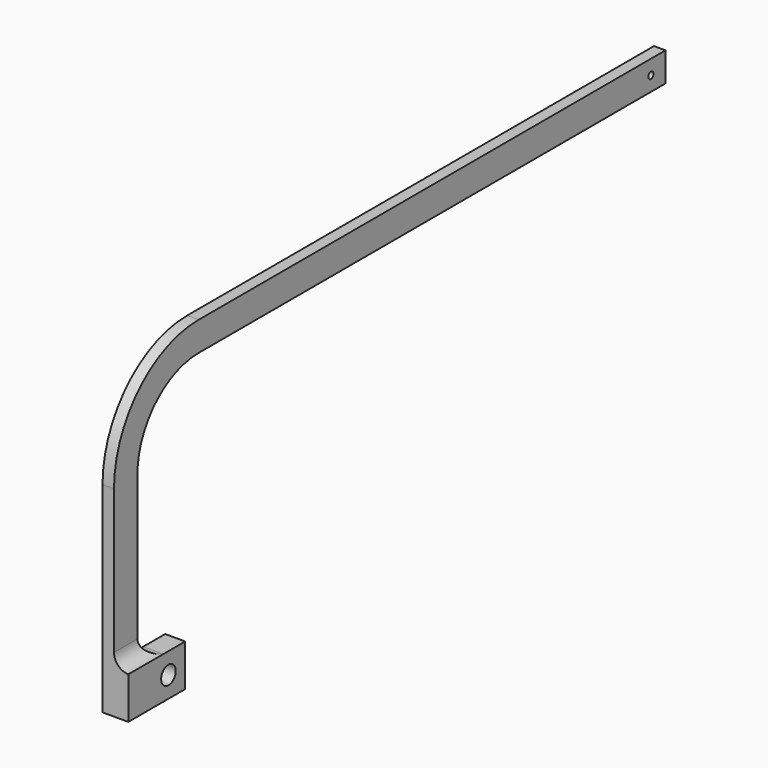
from build123d import *

# Parameters (mm, degrees)
F2_W         = 3.15
F2_H         = 8
F4_W         = 5.5
F4_H         = 19.5
F5_DEPTH     = 11.5
F6_R         = 2.5
F7_DEPTH     = 5.5
F8_T1_DEPTH  = 1.575
F8_T6_DEPTH  = 8
F8_T12_DEPTH = 18
F8_T17_DEPTH = 11.575
F9_R         = 0.9
F10_DEPTH    = 3.15


# Not quite as in the source:
# - a fillet or chamfer that OpenCascade refuses, or shapes differently, is made with other operations: its cross-section is extruded or revolved along the edge and cut away or added


with BuildPart() as f3:
    # F3: sweep along a path in F1
    with BuildLine(Plane.YZ) as f3_path:
        Line((0, 0), (-160, 0))
        ThreePointArc((-160, 0), (-177.6776695297, -7.3223304703), (-185, -25))
        Line((-185, -25), (-185, -80))
    # F2 (on Front) → F3 (sweep)
    with BuildSketch(Plane.XZ):
        Rectangle(F2_W, F2_H)
    sweep(path=f3_path.line)

    # F4 (on face) → F5 (join)
    with BuildSketch(Plane(origin=(0, 0, -80), x_dir=(1, 0, 0), z_dir=(0, 0, -1))):
        with Locations((2.75, 179.25)):
            Rectangle(F4_W, F4_H)
    extrude(amount=-F5_DEPTH)

    # F6 (on face) → F7 (cut, through all)
    with BuildSketch(Plane.YZ.offset(5.5)):
        with Locations((-175.25, -74.25)):
            Circle(F6_R)
    extrude(amount=-F7_DEPTH, mode=Mode.SUBTRACT)

    # F8: fillet of radius 4 on 2 edges, made by hand

    # F8_s2 → F8_t1 (join)
    with BuildSketch(Plane.YZ):
        with BuildLine():
            ThreePointArc((-181, -64.5), (-179.8284271247, -67.3284271247), (-177, -68.5))
            Line((-177, -68.5), (-181, -68.5))
            Line((-181, -68.5), (-181, -64.5))
        make_face()
    extrude(amount=F8_T1_DEPTH)


with BuildPart() as f8_tool4:
    # F8_s5 → F8_t6 (new body)
    with BuildSketch(Plane.XZ.offset(189)):
        with BuildLine():
            ThreePointArc((1.575, -64.5), (2.7465728753, -67.3284271247), (5.575, -68.5))
            Line((5.575, -68.5), (1.575, -68.5))
            Line((1.575, -68.5), (1.575, -64.5))
        make_face()
    extrude(amount=-F8_T6_DEPTH)

    split(bisect_by=Plane.YZ.offset(5.5), keep=Keep.BOTTOM)


with BuildPart() as f3_1:
    add(f3.part)

    # F8_t3: union F8_tool4
    add(f8_tool4.part)


with BuildPart() as f8_tool10:
    # F8_s11 → F8_t12 (new body)
    with BuildSketch(Plane.XZ.offset(189)):
        with BuildLine():
            ThreePointArc((1.575, -64.5), (2.7465728753, -67.3284271247), (5.575, -68.5))
            Line((5.575, -68.5), (1.575, -68.5))
            Line((1.575, -68.5), (1.575, -64.5))
        make_face()
    extrude(amount=-F8_T12_DEPTH)

    split(bisect_by=Plane.XZ.offset(181), keep=Keep.BOTTOM)

    split(bisect_by=Plane.YZ.offset(5.5), keep=Keep.BOTTOM)


with BuildPart() as f8_tool15:
    # F8_s16 → F8_t17 (new body)
    with BuildSketch(Plane.YZ.offset(11.575)):
        with BuildLine():
            ThreePointArc((-181, -64.5), (-179.8284271247, -67.3284271247), (-177, -68.5))
            Line((-177, -68.5), (-181, -68.5))
            Line((-181, -68.5), (-181, -64.5))
        make_face()
    extrude(amount=-F8_T17_DEPTH)

    split(bisect_by=Plane.YZ.offset(1.575), keep=Keep.TOP)

    split(bisect_by=Plane.YZ.offset(5.5), keep=Keep.BOTTOM)


with BuildPart() as f8_tool10_1:
    add(f8_tool10.part)

    # F8_t20: intersect F8_tool15
    add(f8_tool15.part, mode=Mode.INTERSECT)


with BuildPart() as f3_2:
    add(f3_1.part)

    # F8_t8: union F8_tool10
    add(f8_tool10_1.part)

    # F9 (on face) → F10 (cut, through all)
    with BuildSketch(Plane.YZ.offset(1.575)):
        with Locations((-5, 0)):
            Circle(F9_R)
    extrude(amount=-F10_DEPTH, mode=Mode.SUBTRACT)


solid = f3_2.part
